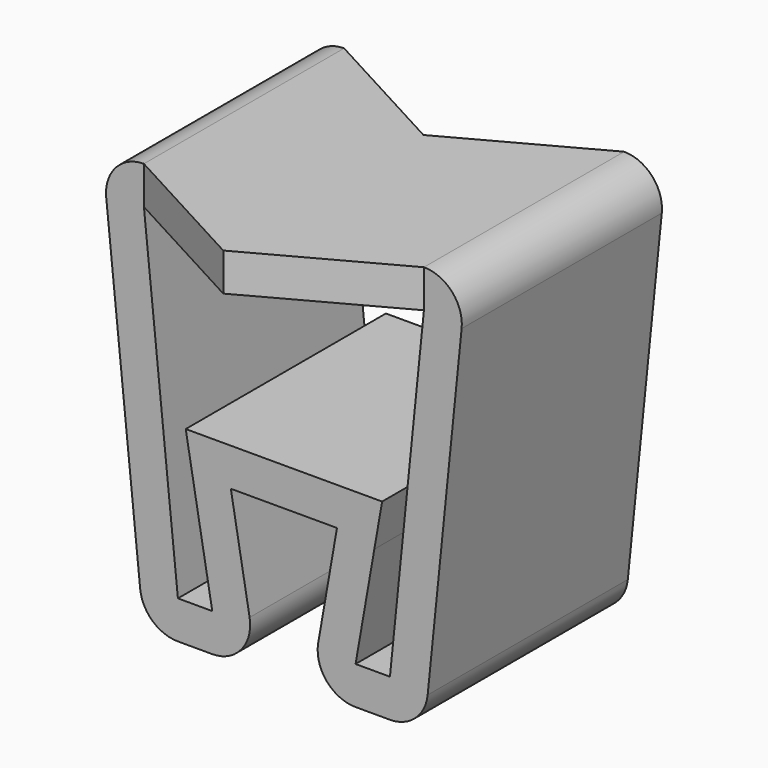
from build123d import *

# Parameters (mm, degrees)
F1_DEPTH    = 3.3
F2_R        = 0.5
F3_T        = 0.5
F3_T3_DEPTH = 4.3
F5_DEPTH    = 0.5
F6_DEPTH    = 0.5


# Not quite as in the source:
# - a shell that OpenCascade refuses in one call is made with other operations: the cavity is built on its own and cut out


with BuildPart() as f1:
    # F0 (on Front) → F1 (new body)
    with BuildSketch(Plane.XZ):
        Polygon((-0.7, -2.4), (0, -2.4), (0.7, -2.4), (0.35, -4.4), (1.85, -4.4), (2.4, 1), (0, 1), (-2.4, 1), (-1.85, -4.4), (-0.35, -4.4), align=None)
    extrude(amount=F1_DEPTH)

    # F2
    f2_edges = [f1.edges().sort_by_distance(p)[0] for p in [
        (2.4, -1.65, 1),
        (1.85, -1.65, -4.4),
        (-0.35, -1.65, -4.4),
        (-2.4, -1.65, 1),
        (0.35, -1.65, -4.4),
        (-1.85, -1.65, -4.4),
    ]]
    fillet(f2_edges, radius=F2_R)

    # F3: shell of thickness 0.5, made by hand


with BuildPart() as f3_core1:
    # F3_t2: copy of F1
    add(f1.part)

    # the walls: a layer under each face that stays
    f3_faces = [f3_core1.faces().sort_by_distance(p)[0] for p in [
        (0.5762916395, -1.65, -3.1069049171),
        (0, -1.65, -2.4),
        (1.17171884, -1.65, -4.4),
        (-0.5762916395, -1.65, -3.1069049171),
        (2.1198397965, -1.65, -1.7506638158),
        (-1.17171884, -1.65, -4.4),
        (0, -1.65, 1),
        (-2.1198397965, -1.65, -1.7506638158),
    ]]
    thicken(f3_faces, amount=-F3_T, mode=Mode.SUBTRACT)

    # F3_s4 → F3_t3 (cut)
    with BuildSketch(Plane.XZ.offset(-0.5)):
        Polygon((0.6950748477, -2.4041380983), (1.1925152336, -2.4861901659), (1.2950985126, -1.9), (0.7, -1.9), align=None)
        Polygon((-0.6950748477, -2.4041380983), (-0.7, -1.9), (-1.2950985126, -1.9), (-1.1925152336, -2.4861901659), align=None)
    extrude(amount=F3_T3_DEPTH, mode=Mode.SUBTRACT)


with BuildPart() as f1_1:
    add(f1.part)

    # what is left inside the walls is the cavity
    f3_cavity = [f3_core1.part.solids().sort_by_distance(p)[0] for p in [
        (-1.617439, -2.2, -1.699493),
    ]]
    add(f3_cavity, mode=Mode.SUBTRACT)

    # F4 (on face) → F5 (join, through all)
    with BuildSketch(Plane.XY.offset(1)):
        Polygon((1.8464873155, -3.3), (-1.8464873155, -3.3), (0, -4.3), align=None)
    extrude(amount=-F5_DEPTH)

    # F4 (on face) → F6 (cut, through all)
    with BuildSketch(Plane.XY.offset(1)):
        Polygon((1.8464873155, 0), (-1.8464873155, 0), (0, -1), align=None)
    extrude(amount=-F6_DEPTH, mode=Mode.SUBTRACT)


solid = f1_1.part
